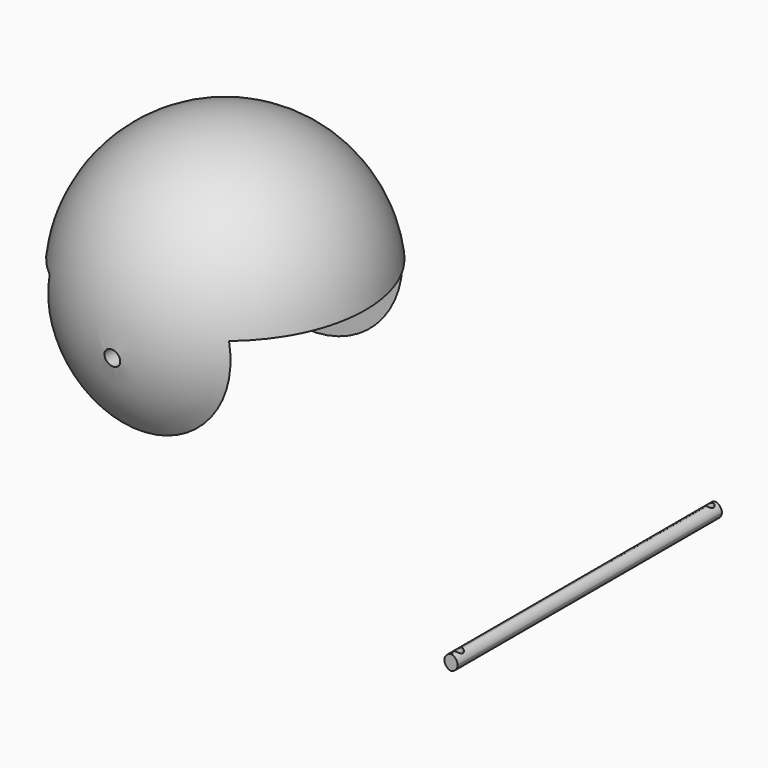
from build123d import *

# Parameters (mm, degrees)
F2_W          = 2301.2386262417
F2_H          = 967.4595296383
F3_DEPTH      = 508
F3_DEPTH_BACK = 508
F4_W          = 1560.4499578476
F4_H          = 71.9765424728
F5_DEPTH      = 63.5
F6_R          = 37.4122033976
F7_DEPTH      = 952.5
F8_R          = 17.3919576193
F8_R_2        = 18.9277654493
F9_DEPTH      = 254
F10_T1_DEPTH  = 1750.9499578476


# Not quite as in the source:
# - a fillet or chamfer that OpenCascade refuses, or shapes differently, is made with other operations: its cross-section is extruded or revolved along the edge and cut away or added


with BuildPart() as f1:
    # F0 (on Front) → F1 (revolve)
    with BuildSketch(Plane.XZ):
        with BuildLine():
            Line((-1699.5742321014, -382.4223577976), (-1033.4309780598, -382.4223577976))
            ThreePointArc((-1033.4309780598, -382.4223577976), (-1699.5742321014, 283.720896244), (-2365.7174861431, -382.4223577976))
            Line((-2365.7174861431, -382.4223577976), (-1699.5742321014, -382.4223577976))
        make_face()
    revolve(axis=Axis((-1366.5026050806, 0, -382.4223577976), (1, 0, 0)))

    # F2 (on Front) → F3 (cut, two sides)
    with BuildSketch(Plane.XZ) as f3_sk:
        with Locations((-1639.2507106066, -788.0810052156)):
            Rectangle(F2_W, F2_H)
    extrude(amount=-F3_DEPTH, mode=Mode.SUBTRACT)
    extrude(f3_sk.sketch, amount=F3_DEPTH_BACK, mode=Mode.SUBTRACT)

    # F6 (on Front) → F7 (cut, symmetric)
    with BuildSketch(Plane.XZ):
        with Locations((-1704.3237686157, -451.4649510384)):
            Circle(F6_R)
    extrude(amount=F7_DEPTH, both=True, mode=Mode.SUBTRACT)


with BuildPart() as f5:
    # F4 (on Right) → F5 (new body)
    with BuildSketch(Plane.YZ):
        with Locations((-51.1900186539, -1084.8415493965)):
            Rectangle(F4_W, F4_H)
    extrude(amount=F5_DEPTH)

    # F8 (on face) → F9 (cut)
    with BuildSketch(Plane.XY.offset(-1048.8532781601)):
        with Locations((31.75, 698.3098983765)):
            Circle(F8_R)
        with Locations((31.75, -785.3997945786)):
            Circle(F8_R_2)
    extrude(amount=-F9_DEPTH, mode=Mode.SUBTRACT)

    # F10: fillet of radius 38.1 on 4 edges, made by hand

    # F10_s2 → F10_t1 (cut)
    with BuildSketch(Plane.XZ.offset(-824.2849602699)):
        with BuildLine():
            ThreePointArc((25.4, -1048.8532781601), (52.3407683632, -1060.0125097969), (63.5, -1086.9532781601))
            Line((63.5, -1086.9532781601), (63.5, -1048.8532781601))
            Line((63.5, -1048.8532781601), (25.4, -1048.8532781601))
        make_face()
        with BuildLine():
            ThreePointArc((63.5, -1082.7298206329), (52.3407683632, -1109.6705889961), (25.4, -1120.8298206329))
            Line((25.4, -1120.8298206329), (63.5, -1120.8298206329))
            Line((63.5, -1120.8298206329), (63.5, -1082.7298206329))
        make_face()
        with BuildLine():
            ThreePointArc((0, -1082.7298206329), (11.1592316368, -1109.6705889961), (38.1, -1120.8298206329))
            Line((38.1, -1120.8298206329), (0, -1120.8298206329))
            Line((0, -1120.8298206329), (0, -1082.7298206329))
        make_face()
        with BuildLine():
            ThreePointArc((38.1, -1048.8532781601), (11.1592316368, -1060.0125097969), (0, -1086.9532781601))
            Line((0, -1086.9532781601), (0, -1048.8532781601))
            Line((0, -1048.8532781601), (38.1, -1048.8532781601))
        make_face()
    extrude(amount=F10_T1_DEPTH, mode=Mode.SUBTRACT)


solid = Compound([f1.part, f5.part])
